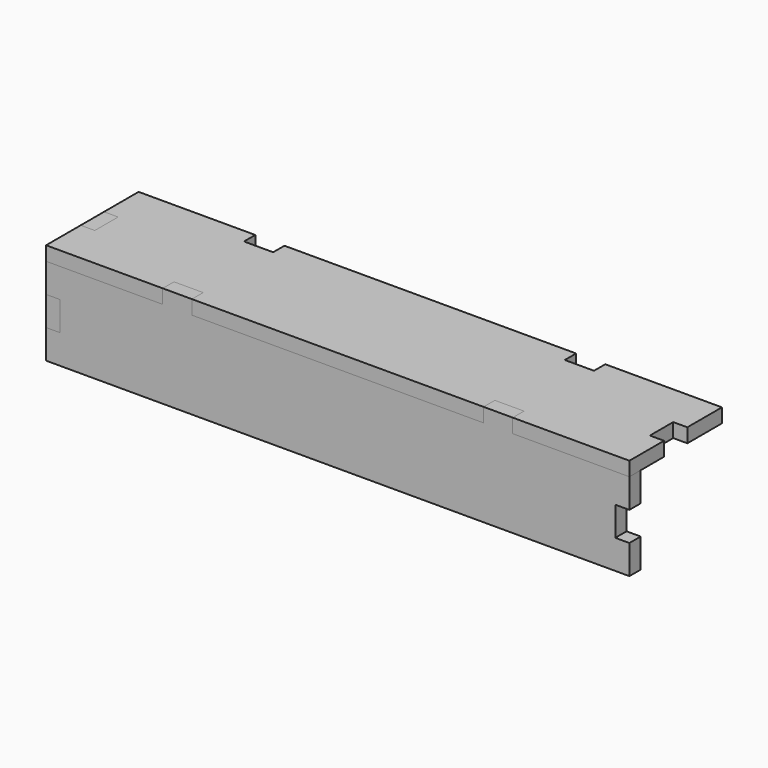
from build123d import *

# Parameters (mm, degrees)
F2_DEPTH = 3.0734
F3_W     = 63.5
F3_H     = 3.0734
F4_DEPTH = 3.0734
F5_W     = 3.0734
F5_H     = 6.35
F6_DEPTH = 3.0734


# Not quite as in the source:
# - a variable given as a bare number and used for a length is read in inches; the dataset says mm whatever the document's units were


with BuildPart() as f2:
    # F1 (on Front) → F2 (new body)
    with BuildSketch(Plane.XZ):
        Polygon((0, 6.35), (0, 0), (127, 0), (127, 6.35), (123.9266, 6.35), (123.9266, 12.7), (127, 12.7), (127, 19.05), (101.6, 19.05), (101.6, 22.1234), (95.25, 22.1234), (95.25, 19.05), (31.75, 19.05), (31.75, 22.1234), (25.4, 22.1234), (25.4, 19.05), (0, 19.05), (0, 12.7), (3.0734, 12.7), (3.0734, 6.35), align=None)
    extrude(amount=-F2_DEPTH)


with BuildPart() as f4:
    # F3 (on face) → F4 (new body)
    with BuildSketch(Plane.XY.offset(19.05)):
        Polygon((0, 0), (25.4, 0), (25.4, 3.0734), (31.75, 3.0734), (95.25, 3.0734), (101.6, 3.0734), (101.6, 0), (127, 0), (127, 9.414411702), (123.9266, 9.414411702), (123.9266, 15.764411702), (127, 15.764411702), (127, 25.178823404), (101.6, 25.178823404), (101.6, 22.105423404), (95.25, 22.105423404), (95.25, 25.178823404), (31.75, 25.178823404), (31.75, 22.105423404), (25.4, 22.105423404), (25.4, 25.178823404), (0, 25.178823404), (0, 15.764411702), (3.0734, 15.764411702), (3.0734, 9.414411702), (0, 9.414411702), align=None)
        with Locations((63.5, 1.5367)):
            Rectangle(F3_W, F3_H)
    extrude(amount=F4_DEPTH)


with BuildPart() as f6:
    # F5 (on face) → F6 (new body)
    with BuildSketch(Plane(origin=(3.0734, 0, 0), x_dir=(0, -1, 0), z_dir=(-1, 0, 0))):
        Polygon((-3.0734, 0), (-3.0734, 6.35), (-3.0734, 12.7), (-3.0734, 19.05), (-9.414411702, 19.05), (-9.414411702, 22.1234), (-15.764411702, 22.1234), (-15.764411702, 19.05), (-22.105423404, 19.05), (-22.105423404, 12.7), (-25.178823404, 12.7), (-25.178823404, 6.35), (-22.105423404, 6.35), (-22.105423404, 0), align=None)
        with Locations((-1.5367, 9.525)):
            Rectangle(F5_W, F5_H)
    extrude(amount=F6_DEPTH)


solid = Compound([f2.part, f4.part, f6.part])
